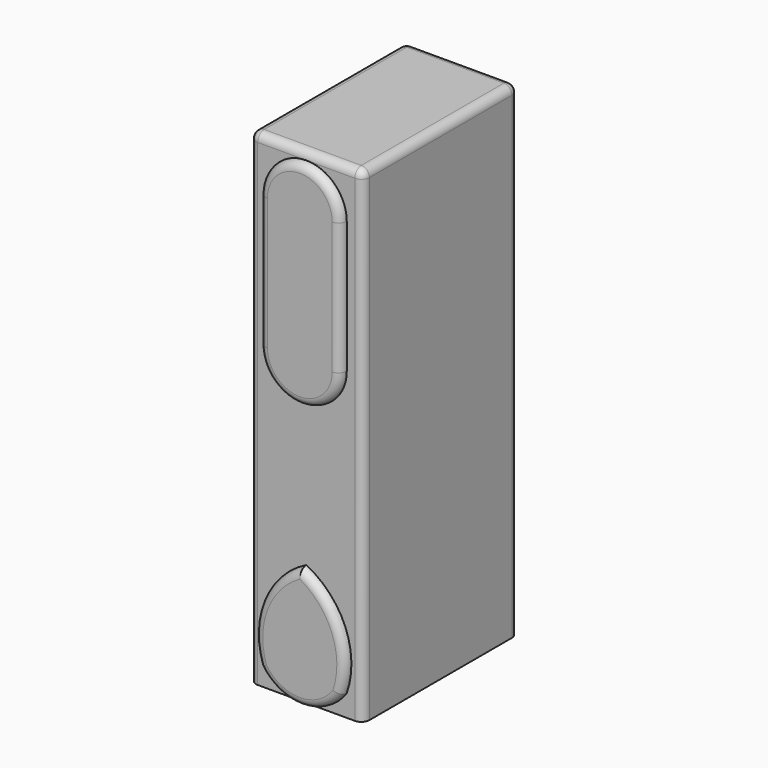
from build123d import *

# Parameters (mm, degrees)
F0_W         = 177.8
F0_H         = 304.8
F1_DEPTH     = 762
F3_DEPTH     = 12.7
F5_T1_DEPTH  = 279.4
F5_T3_DEPTH  = 152.4
F5_T5_DEPTH  = 781.05
F5_T7_DEPTH  = 206.9983323097
F5_S11_W     = 12.954
F5_S11_H     = 12.954
F5_T12_DEPTH = 12.954
F5_S17_W     = 12.954
F5_S17_H     = 12.954
F5_T18_DEPTH = 12.954
F5_S23_W     = 12.954
F5_S23_H     = 12.954
F5_T24_DEPTH = 12.954
F5_S29_W     = 12.954
F5_S29_H     = 12.954
F5_T30_DEPTH = 12.954
F5_T34_ANGLE = 180
F5_T36_ANGLE = 180
F5_T38_ANGLE = 160.6620429302
F5_T40_ANGLE = 121.9975948725
F5_T42_ANGLE = 121.9975948725


# Not quite as in the source:
# - a fillet or chamfer that OpenCascade refuses, or shapes differently, is made with other operations: its cross-section is extruded or revolved along the edge and cut away or added
# - a feature of the source that left no trace in its solid (it failed there, or was rolled back) is left out


with BuildPart() as f1:
    # F0 (on Top) → F1 (new body)
    with BuildSketch(Plane.XY):
        Rectangle(F0_W, F0_H)
    extrude(amount=F1_DEPTH)

    # F2 (on face) → F3 (join)
    with BuildSketch(Plane.XZ.offset(152.4)):
        with BuildLine():
            ThreePointArc((0, 190.5), (-61.5022268, 124.3675088832), (-63.5, 34.0788651625))
            ThreePointArc((-63.5, 34.0788651625), (-36.0333838653, 9.0580961901), (3.12e-07, 0))
            ThreePointArc((3.12e-07, 0), (36.0333841402, 9.0580963377), (63.5, 34.0788651625))
            ThreePointArc((63.5, 34.0788651625), (61.5022268, 124.3675088832), (0, 190.5))
        make_face()
        with BuildLine():
            ThreePointArc((63.5, 685.8), (0, 749.3), (-63.5, 685.8))
            Line((-63.5, 685.8), (-63.5, 478.8016676903))
            ThreePointArc((-63.5, 478.8016676903), (0, 415.3016676903), (63.5, 478.8016676903))
            Line((63.5, 478.8016676903), (63.5, 685.8))
        make_face()
    extrude(amount=F3_DEPTH)

    # F5: fillet of radius 12.7 on 15 edges, made by hand

    # F5_s2 → F5_t1 (cut)
    with BuildSketch(Plane.XZ.offset(-139.7)):
        with BuildLine():
            ThreePointArc((88.9, 749.3), (85.1802561211, 758.2802561211), (76.2, 762))
            Line((76.2, 762), (88.9, 762))
            Line((88.9, 762), (88.9, 749.3))
        make_face()
        with BuildLine():
            ThreePointArc((-76.2, 762), (-85.1802561211, 758.2802561211), (-88.9, 749.3))
            Line((-88.9, 749.3), (-88.9, 762))
            Line((-88.9, 762), (-76.2, 762))
        make_face()
    extrude(amount=F5_T1_DEPTH, mode=Mode.SUBTRACT)

    # F5_s4 → F5_t3 (cut)
    with BuildSketch(Plane.YZ.offset(-76.2)):
        with BuildLine():
            ThreePointArc((152.4, 749.3), (148.6802561211, 758.2802561211), (139.7, 762))
            Line((139.7, 762), (152.4, 762))
            Line((152.4, 762), (152.4, 749.3))
        make_face()
        with BuildLine():
            ThreePointArc((-152.4, 749.3), (-148.6802561211, 758.2802561211), (-139.7, 762))
            Line((-139.7, 762), (-152.4, 762))
            Line((-152.4, 762), (-152.4, 749.3))
        make_face()
    extrude(amount=F5_T3_DEPTH, mode=Mode.SUBTRACT)

    # F5_s6 → F5_t5 (cut)
    with BuildSketch(Plane.XY.offset(-31.75)):
        with BuildLine():
            ThreePointArc((-76.2, -152.4), (-85.1802561211, -148.6802561211), (-88.9, -139.7))
            Line((-88.9, -139.7), (-88.9, -152.4))
            Line((-88.9, -152.4), (-76.2, -152.4))
        make_face()
        with BuildLine():
            ThreePointArc((-76.2, 152.4), (-85.1802561211, 148.6802561211), (-88.9, 139.7))
            Line((-88.9, 139.7), (-88.9, 152.4))
            Line((-88.9, 152.4), (-76.2, 152.4))
        make_face()
        with BuildLine():
            ThreePointArc((88.9, -139.7), (85.1802561211, -148.6802561211), (76.2, -152.4))
            Line((76.2, -152.4), (88.9, -152.4))
            Line((88.9, -152.4), (88.9, -139.7))
        make_face()
        with BuildLine():
            ThreePointArc((88.9, 139.7), (85.1802561211, 148.6802561211), (76.2, 152.4))
            Line((76.2, 152.4), (88.9, 152.4))
            Line((88.9, 152.4), (88.9, 139.7))
        make_face()
    extrude(amount=F5_T5_DEPTH, mode=Mode.SUBTRACT)

    # F5_s8 → F5_t7 (cut)
    with BuildSketch(Plane.XY.offset(478.8016676903)):
        with BuildLine():
            ThreePointArc((63.5, -152.4), (59.7802561211, -161.3802561211), (50.8, -165.1))
            Line((50.8, -165.1), (63.5, -165.1))
            Line((63.5, -165.1), (63.5, -152.4))
        make_face()
        with BuildLine():
            ThreePointArc((-63.5, -152.4), (-59.7802561211, -161.3802561211), (-50.8, -165.1))
            Line((-50.8, -165.1), (-63.5, -165.1))
            Line((-63.5, -165.1), (-63.5, -152.4))
        make_face()
    extrude(amount=F5_T7_DEPTH, mode=Mode.SUBTRACT)


with BuildPart() as f5_tool10:
    # F5_s11 → F5_t12 (new body)
    with BuildSketch(Plane.YZ.offset(76.2)):
        with Locations((-146.177, 755.777)):
            Rectangle(F5_S11_W, F5_S11_H)
    extrude(amount=F5_T12_DEPTH)

    # F5_s13 → F5_t14 (revolve, cut)
    with BuildSketch(Plane(origin=(76.2, -139.7, 749.3), x_dir=(0, 0.7071067812, -0.7071067812), z_dir=(0, -0.7071067812, -0.7071067812))):
        with BuildLine():
            ThreePointArc((0, -12.7), (12.7, 0), (0, 12.7))
            Line((0, 12.7), (0, -12.7))
        make_face()
    revolve(axis=Axis((76.2, -139.7, 749.3), (1, 0, 0)), mode=Mode.SUBTRACT)


with BuildPart() as f1_1:
    add(f1.part)

    # F5_t9: cut F5_tool10
    add(f5_tool10.part, mode=Mode.SUBTRACT)


with BuildPart() as f5_tool16:
    # F5_s17 → F5_t18 (new body)
    with BuildSketch(Plane.YZ.offset(76.2)):
        with Locations((146.177, 755.777)):
            Rectangle(F5_S17_W, F5_S17_H)
    extrude(amount=F5_T18_DEPTH)

    # F5_s19 → F5_t20 (revolve, cut)
    with BuildSketch(Plane(origin=(76.2, 139.7, 749.3), x_dir=(0, -0.7071067812, -0.7071067812), z_dir=(0, -0.7071067812, 0.7071067812))):
        with BuildLine():
            ThreePointArc((0, -12.7), (12.7, 0), (0, 12.7))
            Line((0, 12.7), (0, -12.7))
        make_face()
    revolve(axis=Axis((76.2, 139.7, 749.3), (1, 0, 0)), mode=Mode.SUBTRACT)


with BuildPart() as f1_2:
    add(f1_1.part)

    # F5_t15: cut F5_tool16
    add(f5_tool16.part, mode=Mode.SUBTRACT)


with BuildPart() as f5_tool22:
    # F5_s23 → F5_t24 (new body)
    with BuildSketch(Plane.XZ.offset(-139.7)):
        with Locations((-82.677, 755.777)):
            Rectangle(F5_S23_W, F5_S23_H)
    extrude(amount=-F5_T24_DEPTH)

    # F5_s25 → F5_t26 (revolve, cut)
    with BuildSketch(Plane(origin=(-76.2, 139.7, 749.3), x_dir=(0.7071067812, 0, -0.7071067812), z_dir=(0.7071067812, 0, 0.7071067812))):
        with BuildLine():
            ThreePointArc((0, -12.7), (12.7, 0), (0, 12.7))
            Line((0, 12.7), (0, -12.7))
        make_face()
    revolve(axis=Axis((-76.2, 139.7, 749.3), (0, 1, 0)), mode=Mode.SUBTRACT)


with BuildPart() as f1_3:
    add(f1_2.part)

    # F5_t21: cut F5_tool22
    add(f5_tool22.part, mode=Mode.SUBTRACT)


with BuildPart() as f5_tool28:
    # F5_s29 → F5_t30 (new body)
    with BuildSketch(Plane.XZ.offset(139.7)):
        with Locations((-82.677, 755.777)):
            Rectangle(F5_S29_W, F5_S29_H)
    extrude(amount=F5_T30_DEPTH)

    # F5_s31 → F5_t32 (revolve, cut)
    with BuildSketch(Plane(origin=(-76.2, -139.7, 749.3), x_dir=(0.7071067812, 0, -0.7071067812), z_dir=(-0.7071067812, 0, -0.7071067812))):
        with BuildLine():
            ThreePointArc((0, -12.7), (12.7, 0), (0, 12.7))
            Line((0, 12.7), (0, -12.7))
        make_face()
    revolve(axis=Axis((-76.2, -139.7, 749.3), (0, -1, 0)), mode=Mode.SUBTRACT)


with BuildPart() as f1_4:
    add(f1_3.part)

    # F5_t27: cut F5_tool28
    add(f5_tool28.part, mode=Mode.SUBTRACT)

    # F5_s33 → F5_t34 (revolve, cut)
    with BuildSketch(Plane.XY.offset(478.8016676903)):
        with BuildLine():
            ThreePointArc((-63.5, -152.4), (-59.7802561211, -161.3802561211), (-50.8, -165.1))
            Line((-50.8, -165.1), (-63.5, -165.1))
            Line((-63.5, -165.1), (-63.5, -152.4))
        make_face()
    revolve(axis=Axis((0, -165.1, 478.8016676903), (0, -1, 0)), revolution_arc=F5_T34_ANGLE, mode=Mode.SUBTRACT)

    # F5_s35 → F5_t36 (revolve, cut)
    with BuildSketch(Plane.XY.offset(685.8)):
        with BuildLine():
            ThreePointArc((63.5, -152.4), (59.7802561211, -161.3802561211), (50.8, -165.1))
            Line((50.8, -165.1), (63.5, -165.1))
            Line((63.5, -165.1), (63.5, -152.4))
        make_face()
    revolve(axis=Axis((0, -165.1, 685.8), (0, -1, 0)), revolution_arc=F5_T36_ANGLE, mode=Mode.SUBTRACT)

    # F5_s37 → F5_t38 (revolve, cut)
    with BuildSketch(Plane(origin=(-12.6164174444, 0, 74.050466073), x_dir=(0, 1, 0), z_dir=(-0.1679556687, 0, 0.9857945493))):
        with BuildLine():
            ThreePointArc((-152.4, 63.401778044), (-161.3802561211, 59.6820341651), (-165.1, 50.701778044))
            Line((-165.1, 50.701778044), (-165.1, 63.401778044))
            Line((-165.1, 63.401778044), (-152.4, 63.401778044))
        make_face()
    revolve(axis=Axis((0, -165.1, 76.2), (0, -1, 0)), revolution_arc=F5_T38_ANGLE, mode=Mode.SUBTRACT)

    # F5_s39 → F5_t40 (revolve, cut)
    with BuildSketch(Plane(origin=(69.2556243915, 0, 14.6214058217), x_dir=(0, 1, 0), z_dir=(0.9784320741, 0, 0.2065688173))):
        with BuildLine():
            ThreePointArc((-152.4, 190.3421366621), (-161.3802561211, 186.6223927832), (-165.1, 177.6421366621))
            Line((-165.1, 177.6421366621), (-165.1, 190.3421366621))
            Line((-165.1, 190.3421366621), (-152.4, 190.3421366621))
        make_face()
    revolve(axis=Axis((56.1711141332, -165.1, 76.5973839763), (0, -1, 0)), revolution_arc=F5_T40_ANGLE, mode=Mode.SUBTRACT)

    # F5_s41 → F5_t42 (revolve, cut)
    with BuildSketch(Plane(origin=(11.2454514703, 0, 11.6780216132), x_dir=(0, 1, 0), z_dir=(-0.6936400605, 0, -0.7203217798))):
        with BuildLine():
            ThreePointArc((-152.4, 33.4077090386), (-161.3802561211, 29.6879651596), (-165.1, 20.7077090386))
            Line((-165.1, 20.7077090386), (-165.1, 33.4077090386))
            Line((-165.1, 33.4077090386), (-152.4, 33.4077090386))
        make_face()
    revolve(axis=Axis((-56.1711141332, -165.1, 76.5973839763), (0, -1, 0)), revolution_arc=F5_T42_ANGLE, mode=Mode.SUBTRACT)


solid = f1_4.part
